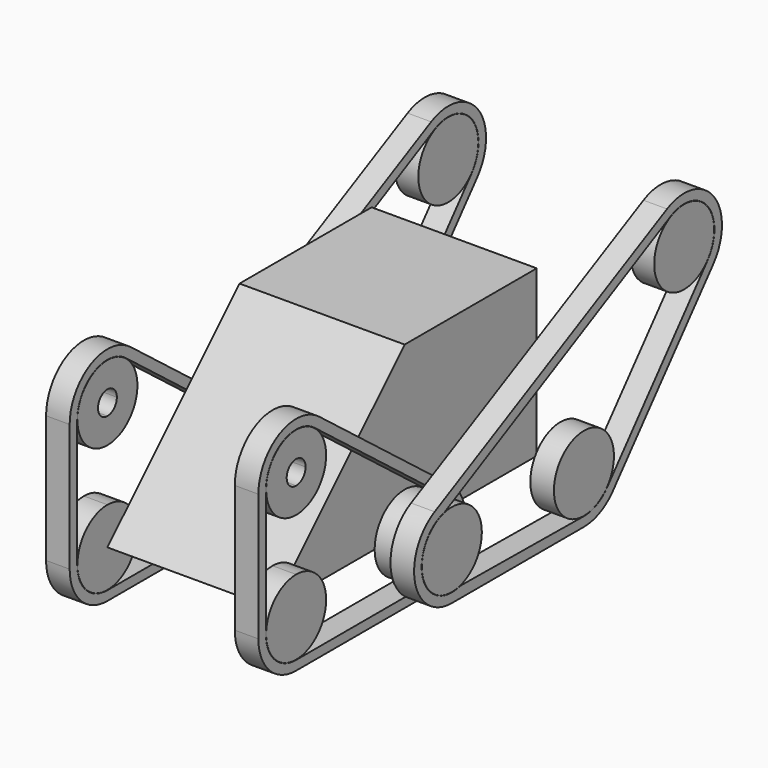
from build123d import *

# Parameters (mm, degrees)
F0_W            = 35
F0_H            = 70
F1_DEPTH        = 35
F3_DEPTH        = 35.001
F5_DEPTH        = 5
F6_DEPTH        = 5
F8_R            = 7.95
F9_DEPTH        = 5
F9_COPIES_COUNT = 2
F9_COPIES_PITCH = 61.032778


# Not quite as in the source:
# - a pattern or mirror of a feature is missing from the dataset's text; its kind, count and spacing are read off the source's solid
# - a feature names something its author has since deleted; it is built from what else it names


with BuildPart() as f1:
    # F0 (on Top) → F1 (new body)
    with BuildSketch(Plane.XY):
        Rectangle(F0_W, F0_H)
    extrude(amount=F1_DEPTH)

    # F2 (on face) → F3 (cut, through all)
    with BuildSketch(Plane.YZ.offset(17.5)):
        Polygon((-35, 0), (0, 35), (-35, 35), align=None)
    extrude(amount=-F3_DEPTH, mode=Mode.SUBTRACT)

    # F4 (on face) → F5 (join)
    with BuildSketch(Plane.YZ.offset(17.5)):
        with BuildLine():
            Line((2.5, 0), (7.95, 0))
            ThreePointArc((7.95, 0), (0, 7.95), (-7.95, 0))
            Line((-7.95, 0), (-2.5, 0))
            ThreePointArc((-2.5, 0), (0, 2.5), (2.5, 0))
        make_face()
        with BuildLine():
            ThreePointArc((-7.95, 0), (0, -7.95), (7.95, 0))
            Line((7.95, 0), (2.5, 0))
            ThreePointArc((2.5, 0), (0, -2.5), (-2.5, 0))
            Line((-2.5, 0), (-7.95, 0))
        make_face()
        with BuildLine():
            Line((-2.5, 0), (2.5, 0))
            ThreePointArc((2.5, 0), (0, 2.5), (-2.5, 0))
        make_face()
        with BuildLine():
            ThreePointArc((-2.5, 0), (0, -2.5), (2.5, 0))
            Line((2.5, 0), (-2.5, 0))
        make_face()
        with BuildLine():
            Line((10, 0), (8, 0))
            ThreePointArc((8, 0), (5.6568542495, -5.6568542495), (0, -8))
            Line((0, -8), (-35, -8))
            ThreePointArc((-35, -8), (-40.6568542495, -5.6568542495), (-43, 0))
            Line((-43, 0), (-43, 27))
            ThreePointArc((-43, 27), (-40.6568542495, 32.6568542495), (-35, 35))
            ThreePointArc((-35, 35), (-32.4187274801, 34.5721220393), (-30.1135723657, 33.3342580445))
            Line((-30.1135723657, 33.3342580445), (-14.0543132631, 20.9456867369))
            Line((-14.0543132631, 20.9456867369), (-12.6283754499, 22.3716245501))
            Line((-12.6283754499, 22.3716245501), (-28.8919654571, 34.9178225556))
            ThreePointArc((-28.8919654571, 34.9178225556), (-39.4113294238, 35.9744176811), (-45, 27))
            Line((-45, 27), (-45, 0))
            ThreePointArc((-45, 0), (-42.0710678119, -7.0710678119), (-35, -10))
            Line((-35, -10), (0, -10))
            ThreePointArc((0, -10), (7.0710678119, -7.0710678119), (10, 0))
        make_face()
        with BuildLine():
            ThreePointArc((4.8864276343, 6.3342580445), (7.1795341449, 3.5290635391), (8, 0))
            Line((8, 0), (10, 0))
            ThreePointArc((10, 0), (8.9744176811, 4.4113294238), (6.1080345429, 7.9178225556))
            Line((6.1080345429, 7.9178225556), (-12.6283754499, 22.3716245501))
            Line((-12.6283754499, 22.3716245501), (-14.0543132631, 20.9456867369))
            Line((-14.0543132631, 20.9456867369), (4.8864276343, 6.3342580445))
        make_face()
        with BuildLine():
            Line((-32.5, 0), (-27.05, 0))
            ThreePointArc((-27.05, 0), (-27.6551577165, 3.0423332873), (-29.3785010896, 5.6214989104))
            Line((-29.3785010896, 5.6214989104), (-33.232233047, 1.767766953))
            ThreePointArc((-33.232233047, 1.767766953), (-32.6903011687, 0.9567085809), (-32.5, 0))
        make_face()
        with BuildLine():
            ThreePointArc((-35, 7.95), (-40.6214989104, -5.6214989104), (-27.05, 0))
            Line((-27.05, 0), (-32.5, 0))
            ThreePointArc((-32.5, 0), (-36.767766953, -1.767766953), (-35, 2.5))
            Line((-35, 2.5), (-35, 7.95))
        make_face()
        with BuildLine():
            Line((-33.232233047, 1.767766953), (-29.3785010896, 5.6214989104))
            ThreePointArc((-29.3785010896, 5.6214989104), (-31.9576667127, 7.3448422835), (-35, 7.95))
            Line((-35, 7.95), (-35, 2.5))
            ThreePointArc((-35, 2.5), (-34.0432914191, 2.3096988313), (-33.232233047, 1.767766953))
        make_face()
        with BuildLine():
            Line((-35, 0), (-32.5, 0))
            ThreePointArc((-32.5, 0), (-32.6903011687, 0.9567085809), (-33.232233047, 1.767766953))
            Line((-33.232233047, 1.767766953), (-35, 0))
        make_face()
        with BuildLine():
            ThreePointArc((-35, 2.5), (-36.767766953, -1.767766953), (-32.5, 0))
            Line((-32.5, 0), (-35, 0))
            Line((-35, 0), (-35, 2.5))
        make_face()
        with BuildLine():
            Line((-35, 0), (-33.232233047, 1.767766953))
            ThreePointArc((-33.232233047, 1.767766953), (-34.0432914191, 2.3096988313), (-35, 2.5))
            Line((-35, 2.5), (-35, 0))
        make_face()
    extrude(amount=F5_DEPTH)

    # F4 (on face) → F6 (join)
    with BuildSketch(Plane.YZ.offset(17.5)):
        with BuildLine():
            Line((6.1080345429, 7.9178225556), (-28.8919654571, 34.9178225556))
            ThreePointArc((-28.8919654571, 34.9178225556), (-39.4113294238, 35.9744176811), (-45, 27))
            Line((-45, 27), (-45, 0))
            ThreePointArc((-45, 0), (-42.0710678119, -7.0710678119), (-35, -10))
            Line((-35, -10), (0, -10))
            ThreePointArc((0, -10), (9.4651525491, -3.2265906499), (6.1080345429, 7.9178225556))
        make_face()
        with BuildLine():
            ThreePointArc((-43, 27), (-38.5290635391, 34.1795341449), (-30.1135723657, 33.3342580445))
            Line((-30.1135723657, 33.3342580445), (4.8864276343, 6.3342580445))
            ThreePointArc((4.8864276343, 6.3342580445), (7.5721220393, -2.5812725199), (0, -8))
            Line((0, -8), (-35, -8))
            ThreePointArc((-35, -8), (-40.6568542495, -5.6568542495), (-43, 0))
            Line((-43, 0), (-43, 27))
        make_face(mode=Mode.SUBTRACT)
    extrude(amount=F6_DEPTH)

    # F7: F1, F5 across plane


with BuildPart() as f5:
    # F4 (on face) → F5, piece 2 (new body)
    with BuildSketch(Plane.YZ.offset(17.5)):
        with BuildLine():
            Line((-35, 24.5), (-35, 19.05))
            ThreePointArc((-35, 19.05), (-29.3785010896, 21.3785010896), (-27.05, 27))
            ThreePointArc((-27.05, 27), (-29.3785010896, 32.6214989104), (-35, 34.95))
            Line((-35, 34.95), (-35, 29.5))
            ThreePointArc((-35, 29.5), (-33.232233047, 28.767766953), (-32.5, 27))
            ThreePointArc((-32.5, 27), (-33.232233047, 25.232233047), (-35, 24.5))
        make_face()
        with BuildLine():
            ThreePointArc((-35, 34.95), (-42.95, 27), (-35, 19.05))
            Line((-35, 19.05), (-35, 24.5))
            ThreePointArc((-35, 24.5), (-37.5, 27), (-35, 29.5))
            Line((-35, 29.5), (-35, 34.95))
        make_face()
    extrude(amount=F5_DEPTH)


with BuildPart() as f1_1:
    add(f1.part)
    add(f1.part.mirror(Plane.YZ))
    add(f5.part.mirror(Plane.YZ))

    # F8 (on face) → F9, piece 3 (join)
    with BuildSketch(Plane.YZ.offset(22.5)):
        with BuildLine():
            Line((57.0210172366, 40.3724198063), (-4.5508668554, 8.9044713972))
            ThreePointArc((-4.5508668554, 8.9044713972), (-9.7222608989, -2.3404365007), (0, -10))
            Line((0, -10), (35, -10))
            ThreePointArc((35, -10), (39.2120901339, -9.0696359742), (42.640424841, -6.4516593408))
            Line((42.640424841, -6.4516593408), (69.2123089329, 25.0162890683))
            ThreePointArc((69.2123089329, 25.0162890683), (69.4038078625, 37.6857430384), (57.0210172366, 40.3724198063))
        make_face()
        with BuildLine():
            ThreePointArc((57.9080220764, 38.5796370363), (67.8293190298, 36.4523749557), (67.6842239647, 26.3066209364))
            Line((67.6842239647, 26.3066209364), (41.1123398728, -5.1613274726))
            ThreePointArc((41.1123398728, -5.1613274726), (38.3333809066, -7.2724529378), (34.920065821, -7.999600648))
            Line((34.920065821, -7.999600648), (2.2629077537, -7.6732814687))
            ThreePointArc((2.2629077537, -7.6732814687), (-7.7262338594, -2.0749241795), (-1.8857040225, 7.7745816826))
            Line((-1.8857040225, 7.7745816826), (57.9080220764, 38.5796370363))
        make_face(mode=Mode.SUBTRACT)
        with BuildLine():
            ThreePointArc((7.95, 0), (4.8280754869, 6.3160262106), (-2.0857703378, 7.6715097665))
            ThreePointArc((-2.0857703378, 7.6715097665), (-7.671510585, -2.0857673274), (2.0857643171, -7.6715114035))
            ThreePointArc((2.0857643171, -7.6715114035), (6.316024316, -4.8280779654), (7.95, 0))
        make_face()
    extrude(amount=F9_DEPTH)

    # F9_copies: F9 ×2


with BuildPart() as f9:
    # F8 (on face) → F9 (new body)
    with BuildSketch(Plane.YZ.offset(22.5)):
        with Locations((35, 0)):
            Circle(F8_R)
    extrude(amount=F9_DEPTH)


with BuildPart() as f9b:
    # F8 (on face) → F9, piece 2 (new body)
    with BuildSketch(Plane.YZ.offset(22.5)):
        with Locations((61.571884092, 31.467948409)):
            Circle(F8_R)
    extrude(amount=F9_DEPTH)


with BuildPart() as f1_2:
    add(f1_1.part)
    with Locations(*[Vector(-0.8192319205, -0.5734623444, 0) * (i * F9_COPIES_PITCH) for i in range(1, F9_COPIES_COUNT)]):
        add(f9.part)



with BuildPart() as f1_3:
    add(f1_2.part)

    add(f5.part)  # F10 merges F5
    # F10: F1, F9, F9b across plane
    add(f1_2.part.mirror(Plane.YZ))
    add(f9.part.mirror(Plane.YZ))
    add(f9b.part.mirror(Plane.YZ))


solid = Compound([f9.part, f9b.part, f1_3.part])
